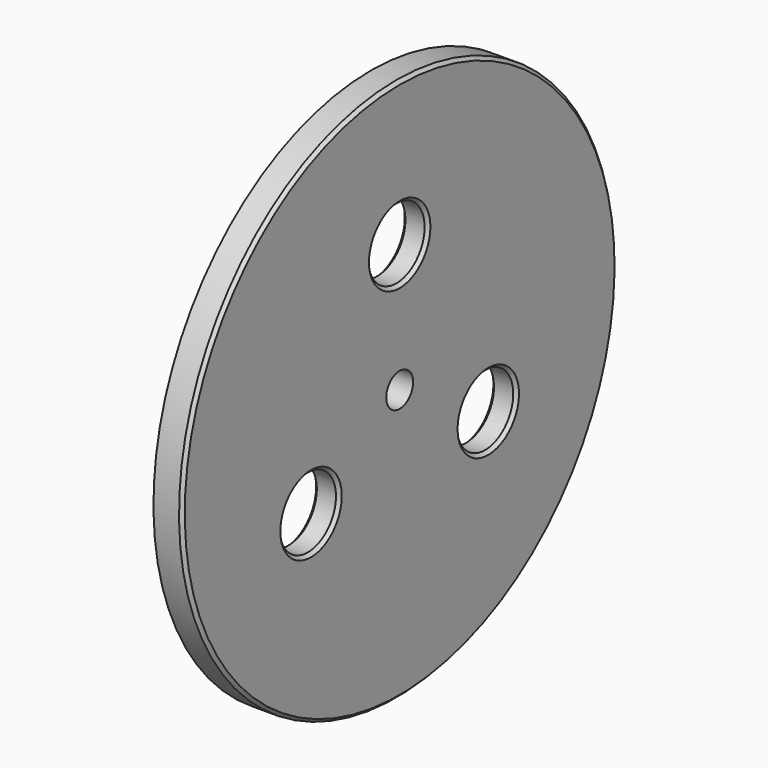
from build123d import *

# Parameters (mm, degrees)
F3_D    = 10.5
F5_D    = 22
F6_SIZE = 1


with BuildPart() as f1:
    # F0 (on Front) → F1 (revolve)
    with BuildSketch(Plane.XZ):
        Polygon((0, 85), (0, 80), (1, 80), (1, 0), (9, 0), (9, 85), align=None)
    revolve(axis=Axis((5, 0, 0), (-1, 0, 0)))

    # F3 (through all)
    with Locations(Plane.YZ.offset(9)):
        with Locations((0, 0)):
            Hole(F3_D / 2)

    # F5 (through all)
    with Locations(Plane.YZ.offset(9)):
        with Locations((0, 40), (34.6410161514, -20), (-34.6410161514, -20)):
            Hole(F5_D / 2)

    # F6
    f6_edges = [f1.edges().sort_by_distance(p)[0] for p in [
        (9, 0, -85),
        (9, -45.641016, -20),
        (9, -11, 40),
        (9, 23.641016, -20),
        (1, -45.641016, -20),
        (1, 23.641016, -20),
        (1, -11, 40),
    ]]
    chamfer(f6_edges, length=F6_SIZE)


solid = f1.part
